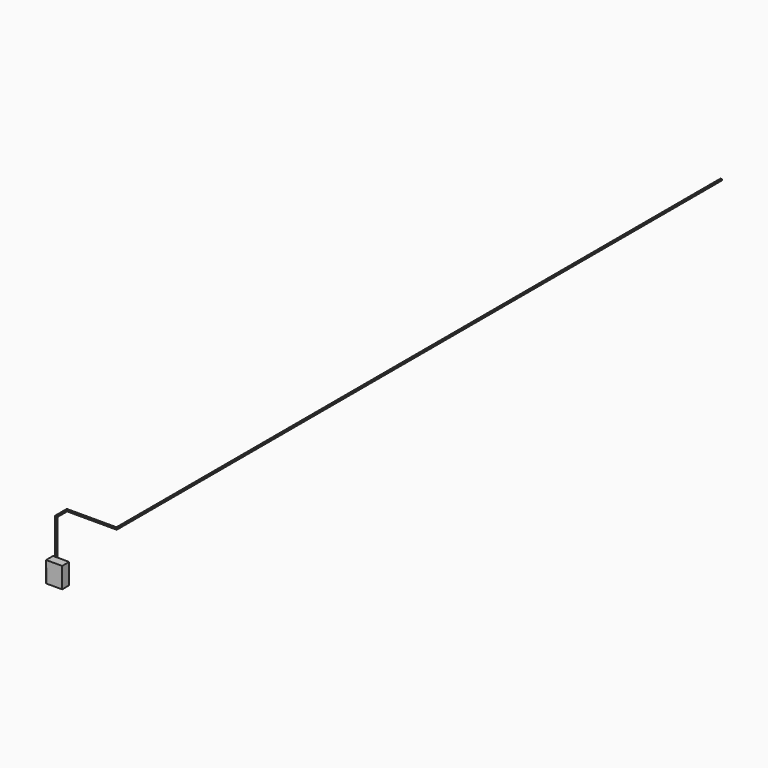
from build123d import *

# Parameters (mm, degrees)
F0_W      = 1778
F0_H      = 965.2
F1_DEPTH  = 2286
F2_W      = 170.18
F2_H      = 127
F3_DEPTH  = 1524
F4_W      = 170.18
F4_H      = 127
F5_DEPTH  = 1219.2
F6_W      = 170.18
F6_H      = 127
F7_DEPTH  = 4572
F8_W      = 170.18
F8_H      = 127
F9_DEPTH  = 1524
F10_W     = 170.18
F10_H     = 127
F11_DEPTH = 5486.4
F12_W     = 170.18
F12_H     = 127
F13_DEPTH = 83515.2


with BuildPart() as f1:
    # F0 (on Top) → F1 (new body)
    with BuildSketch(Plane.XY):
        with Locations((889, 482.6)):
            Rectangle(F0_W, F0_H)
    extrude(amount=F1_DEPTH)


with BuildPart() as f3:
    # F2 (on Top) → F3 (new body)
    with BuildSketch(Plane.XY):
        with Locations((85.09, 63.5)):
            Rectangle(F2_W, F2_H)
    extrude(amount=F3_DEPTH)

    # F4 (on face) → F5 (join)
    with BuildSketch(Plane(origin=(0, 127, 0), x_dir=(-1, 0, 0), z_dir=(0, 1, 0))):
        with Locations((-85.09, 1460.5)):
            Rectangle(F4_W, F4_H)
    extrude(amount=F5_DEPTH)

    # F6 (on face) → F7 (join)
    with BuildSketch(Plane.XY.offset(1524)):
        with Locations((85.09, 1282.7)):
            Rectangle(F6_W, F6_H)
    extrude(amount=F7_DEPTH)

    # F8 (on face) → F9 (join)
    with BuildSketch(Plane(origin=(0, 1346.2, 0), x_dir=(-1, 0, 0), z_dir=(0, 1, 0))):
        with Locations((-85.09, 6032.5)):
            Rectangle(F8_W, F8_H)
    extrude(amount=F9_DEPTH)

    # F10 (on face) → F11 (join)
    with BuildSketch(Plane.YZ.offset(170.18)):
        with Locations((2785.11, 6032.5)):
            Rectangle(F10_W, F10_H)
    extrude(amount=F11_DEPTH)

    # F12 (on face) → F13 (join)
    with BuildSketch(Plane(origin=(0, 2870.2, 0), x_dir=(-1, 0, 0), z_dir=(0, 1, 0))):
        with Locations((-5571.49, 6032.5)):
            Rectangle(F12_W, F12_H)
    extrude(amount=F13_DEPTH)


solid = Compound([f1.part, f3.part])
